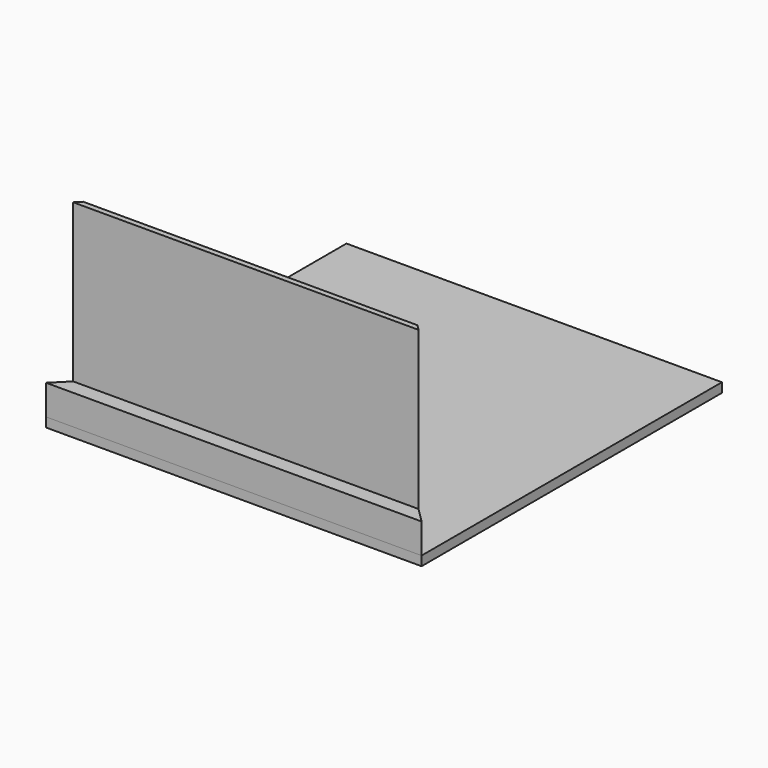
from build123d import *

# Parameters (mm, degrees)
F0_W     = 600
F0_H     = 600
F1_DEPTH = 15
F3_DEPTH = 48
F4_W     = 552
F4_H     = 300
F5_DEPTH = 9
F6_SIZE  = 8.99999


# Not quite as in the source:
# - a fillet or chamfer is up to 0.001 mm smaller than in the source, because OpenCascade refuses the exact size


with BuildPart() as f1:
    # F0 (on Top) → F1 (new body)
    with BuildSketch(Plane.XY):
        Rectangle(F0_W, F0_H)
    extrude(amount=F1_DEPTH)


with BuildPart() as f3:
    # F2 (on face) → F3 (new body)
    with BuildSketch(Plane.XY.offset(15)):
        Polygon((-276, -276), (-300, -300), (300, -300), (276, -276), align=None)
    extrude(amount=F3_DEPTH)


with BuildPart() as f5:
    # F4 (on face) → F5 (new body)
    with BuildSketch(Plane(origin=(0, -276, 0), x_dir=(-1, 0, 0), z_dir=(0, 1, 0))):
        with Locations((0, 165)):
            Rectangle(F4_W, F4_H)
    extrude(amount=F5_DEPTH)

    # F6 (size 9 in the source; OpenCascade refuses exactly that, so slightly less here)
    f6_edges = [f5.edges().sort_by_distance(p)[0] for p in [
        (276, -267, 165),
        (-276, -267, 165),
    ]]
    chamfer(f6_edges, length=F6_SIZE)


solid = Compound([f1.part, f3.part, f5.part])
